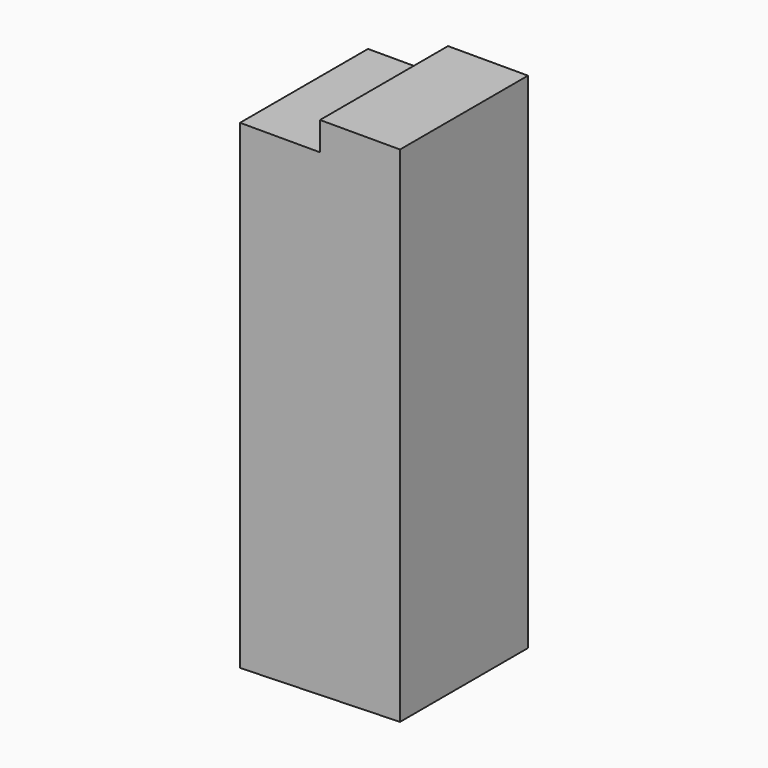
from build123d import *

# Parameters (mm, degrees)
F1_DEPTH = 12.7


# Not quite as in the source:
# - the program builds the solid bodies; features that only make, move or delete a surface that nothing else refers to are left out


with BuildPart() as f1:
    # F0 (on Front) → F1 (new body, symmetric)
    with BuildSketch(Plane.XZ):
        Polygon((-31.9411642849, 34.2251690984), (-31.9411642849, -41.9748309016), (-6.5411642849, -41.2616990507), (-6.5411642849, 38.7482978404), (-19.2411642849, 38.7482978404), (-19.2411642849, 34.2251690984), align=None)
    extrude(amount=F1_DEPTH, both=True)


solid = f1.part
